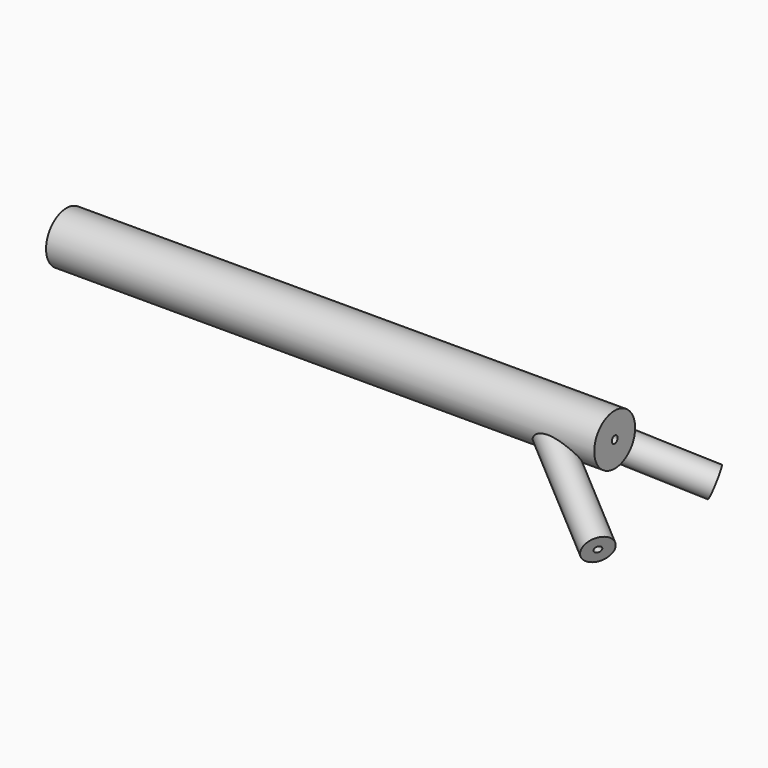
from build123d import *
from build123d import SkipClean  # not in build123d's __all__

# Parameters (mm, degrees)
F0_R      = 7
F1_DEPTH  = 75
F2_R      = 1
F3_DEPTH  = 150.001
F4_R      = 5.5
F4_R_2    = 1
F5_DEPTH  = 8
F6_W      = 0.5
F6_H      = 0.5
F13_R     = 4
F14_DEPTH = 40
F16_R     = 1
F17_DEPTH = 40
F18_R     = 4
F19_DEPTH = 40
F20_R     = 1
F21_DEPTH = 33


with BuildPart() as f1:
    # F0 (on Right) → F1 (new body, symmetric)
    with BuildSketch(Plane.YZ):
        Circle(F0_R)
    extrude(amount=F1_DEPTH, both=True)

    # F2 (on face) → F3 (cut, through all)
    with BuildSketch(Plane(origin=(-75, 0, 0), x_dir=(0, -1, 0), z_dir=(-1, 0, 0))):
        Circle(F2_R)
    extrude(amount=-F3_DEPTH, mode=Mode.SUBTRACT)

    # F4 (on face) → F5 (cut)
    with BuildSketch(Plane(origin=(-75, 0, 0), x_dir=(0, -1, 0), z_dir=(-1, 0, 0))):
        Circle(F4_R)
        Circle(F4_R_2, mode=Mode.SUBTRACT)
    extrude(amount=-F5_DEPTH, mode=Mode.SUBTRACT)

    # F6 (on Top) → F7 (revolve, cut)
    with BuildSketch(Plane.XY):
        with Locations((-66.75, 1.75)):
            Rectangle(F6_W, F6_H)
    revolve(axis=Axis((-60.2624397725, 0, 0), (1, 0, 0)), mode=Mode.SUBTRACT)

    # F13 (on face) → F14 (join)
    with BuildSketch(Plane(origin=(33.8824944498, 21.5843530986, -15.7996666393), x_dir=(-0.4531538935, 0.8660254038, 0.2113091309), z_dir=(0.7848855672, 0.5, -0.3659981508))):
        with Locations((-24.9234641435, 23.2440043957)):
            Circle(F13_R)
    extrude(amount=F14_DEPTH)

    # F16 (on face) → F17 (cut)
    with BuildSketch(Plane(origin=(65.2779171386, 41.5843530986, -30.4395926702), x_dir=(-0.4531538935, 0.8660254038, 0.2113091309), z_dir=(0.7848855672, 0.5, -0.3659981508))):
        with Locations((-24.9234641435, 23.2440043957)):
            Circle(F16_R)
    extrude(amount=-F17_DEPTH, mode=Mode.SUBTRACT)

    # F18 (on face) → F19 (join)
    with BuildSketch(Plane(origin=(33.8824944498, -21.5843530986, -15.7996666393), x_dir=(-0.4531538935, -0.8660254038, 0.2113091309), z_dir=(-0.7848855672, 0.5, 0.3659981508))):
        with Locations((-24.9234641435, 23.2440043957)):
            Circle(F18_R)
    with SkipClean():  # cleaning this boolean's faces spoils the solid; the shape is the same uncleaned
        extrude(amount=-F19_DEPTH)

    # F20 (on face) → F21 (cut)
    with BuildSketch(Plane(origin=(65.2779171386, -41.5843530986, -30.4395926702), x_dir=(0.4531538935, 0.8660254038, -0.2113091309), z_dir=(0.7848855672, -0.5, -0.3659981508))):
        with Locations((24.9234641435, 23.2440043957)):
            Circle(F20_R)
    with SkipClean():  # cleaning this boolean's faces spoils the solid; the shape is the same uncleaned
        extrude(amount=-F21_DEPTH, mode=Mode.SUBTRACT)


solid = f1.part
